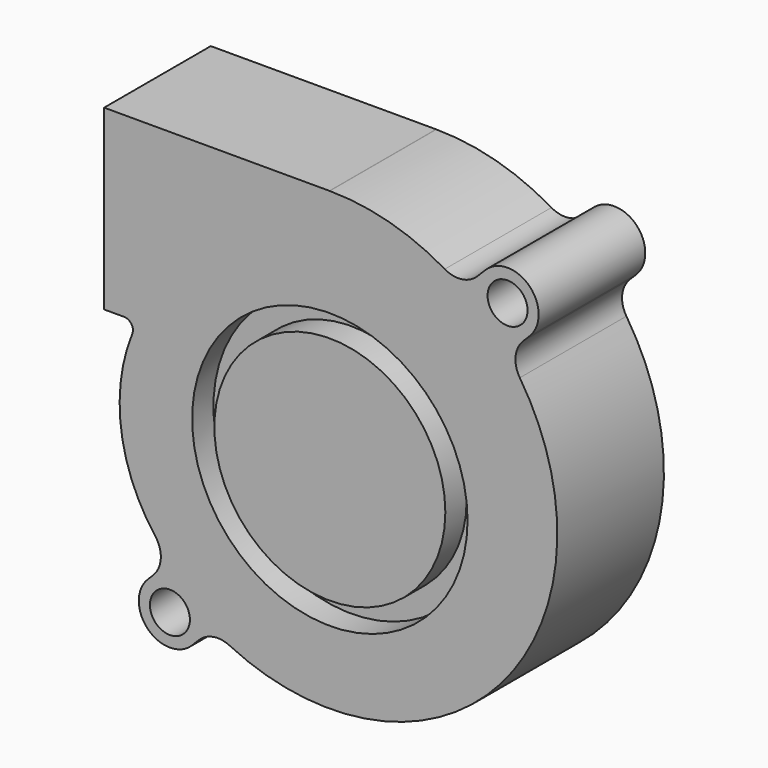
from build123d import *

# Parameters (mm, degrees)
F0_R     = 2.25
F0_R_2   = 15.5
F0_R_3   = 13
F1_DEPTH = 15
F2_DEPTH = 3
F3_W     = 12.2
F3_H     = 17.6
F4_DEPTH = 11.3
F5_R     = 1
F6_R     = 3


# Not quite as in the source:
# - ends of sketch curves that miss each other by under 0.0002 mm in the source are joined


with BuildPart() as f1:
    # F0 (on Front) → F1 (new body)
    with BuildSketch(Plane.XZ):
        with BuildLine():
            Line((-0.05, 27.5966813602), (-25.4, 27.5966813602))
            Line((-25.4, 27.5966813602), (-25.4, 7.5966813602))
            Line((-25.4, 7.5966813602), (-21.614542231, 7.5966813602))
            ThreePointArc((-21.614542231, 7.5966813602), (-23.4006244197, -4.2813010605), (-17.918619958, -14.9688724896))
            Line((-17.918619958, -14.9688724896), (-20.4748737342, -17.5251262658))
            ThreePointArc((-20.4748737342, -17.5251262658), (-20.4748737342, -22.4748737342), (-15.5251262658, -22.4748737342))
            Line((-15.5251262658, -22.4748737342), (-13.153804753, -20.1035522213))
            ThreePointArc((-13.153804753, -20.1035522213), (19.3130689129, -14.8757459996), (19.9528476572, 18.0031001889))
            Line((19.9528476572, 18.0031001889), (22.4748737342, 20.5251262658))
            ThreePointArc((22.4748737342, 20.5251262658), (22.4748737342, 25.4748737342), (17.5251262658, 25.4748737342))
            Line((17.5251262658, 25.4748737342), (14.8648475796, 22.8145950479))
            ThreePointArc((14.8648475796, 22.8145950479), (7.8051661925, 26.3642746914), (-9.5e-08, 27.5966326274))
            Line((-9.5e-08, 27.5966326274), (-0.05, 27.5966813602))
        make_face()
        with Locations((-18, -20)):
            Circle(F0_R, mode=Mode.SUBTRACT)
        Circle(F0_R_2, mode=Mode.SUBTRACT)
        with Locations((20, 23)):
            Circle(F0_R, mode=Mode.SUBTRACT)
        Circle(F0_R_2)
        Circle(F0_R_3, mode=Mode.SUBTRACT)
        Circle(F0_R_3)
    extrude(amount=-F1_DEPTH)

    # F0 (on Front) → F2 (cut)
    with BuildSketch(Plane.XZ):
        Circle(F0_R_2)
        Circle(F0_R_3, mode=Mode.SUBTRACT)
    extrude(amount=-F2_DEPTH, mode=Mode.SUBTRACT)

    # F3 (on face) → F4 (cut)
    with BuildSketch(Plane(origin=(-25.4, 0, 0), x_dir=(0, -1, 0), z_dir=(-1, 0, 0))):
        with Locations((-7.1, 17.5966813602)):
            Rectangle(F3_W, F3_H)
    extrude(amount=-F4_DEPTH, mode=Mode.SUBTRACT)

    # F5
    f5_edges = [f1.edges().sort_by_distance(p)[0] for p in [
        (-21.614542, 7.5, 7.596681),
    ]]
    fillet(f5_edges, radius=F5_R)

    # F6
    f6_edges = [f1.edges().sort_by_distance(p)[0] for p in [
        (-17.91862, 7.5, -14.968872),
        (-13.153805, 7.5, -20.103552),
        (19.952848, 7.5, 18.0031),
        (14.864848, 7.5, 22.814595),
    ]]
    fillet(f6_edges, radius=F6_R)


solid = f1.part
